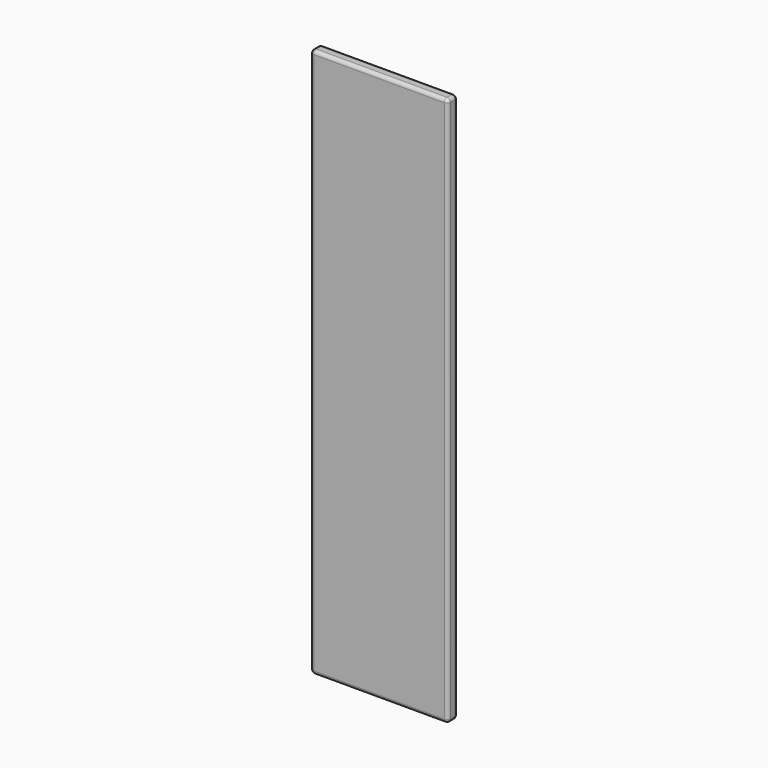
from build123d import *

# Parameters (mm, degrees)
F0_W         = 200
F0_H         = 800
F1_DEPTH     = 18
F2_R         = 5
F3_T1_DEPTH  = 8
F3_S5_W      = 5
F3_S5_H      = 5
F3_T6_DEPTH  = 5
F3_S11_W     = 5
F3_S11_H     = 5
F3_T12_DEPTH = 5


# Not quite as in the source:
# - a fillet or chamfer that OpenCascade refuses, or shapes differently, is made with other operations: its cross-section is extruded or revolved along the edge and cut away or added


with BuildPart() as f1:
    # F0 (on Front) → F1 (new body)
    with BuildSketch(Plane.XZ):
        with Locations((-100, 169.3565798058)):
            Rectangle(F0_W, F0_H)
    extrude(amount=F1_DEPTH)

    # F2
    f2_edges = [f1.edges().sort_by_distance(p)[0] for p in [
        (-200, -18, 169.35658),
        (-200, 0, 169.35658),
        (-100, -18, -230.64342),
        (-100, 0, -230.64342),
        (0, -18, 169.35658),
        (-200, -9, -230.64342),
        (0, -9, -230.64342),
        (-200, -9, 569.35658),
        (-100, -18, 569.35658),
        (-100, 0, 569.35658),
        (0, 0, 169.35658),
    ]]
    fillet(f2_edges, radius=F2_R)

    # F3: fillet of radius 5 on 1 edges, made by hand

    # F3_s2 → F3_t1 (cut)
    with BuildSketch(Plane.XZ.offset(5)):
        with BuildLine():
            ThreePointArc((0, 564.3565798058), (-1.4644660941, 567.8921137117), (-5, 569.3565798058))
            Line((-5, 569.3565798058), (0, 569.3565798058))
            Line((0, 569.3565798058), (0, 564.3565798058))
        make_face()
    extrude(amount=F3_T1_DEPTH, mode=Mode.SUBTRACT)


with BuildPart() as f3_tool4:
    # F3_s5 → F3_t6 (new body)
    with BuildSketch(Plane.YZ.offset(-5)):
        with Locations((-2.5, 566.8565798058)):
            Rectangle(F3_S5_W, F3_S5_H)
    extrude(amount=F3_T6_DEPTH)

    # F3_s7 → F3_t8 (revolve, cut)
    with BuildSketch(Plane(origin=(-5, -5, 564.3565798058), x_dir=(0, -0.7071067812, -0.7071067812), z_dir=(0, -0.7071067812, 0.7071067812))):
        with BuildLine():
            ThreePointArc((0, -5), (5, 0), (0, 5))
            Line((0, 5), (0, -5))
        make_face()
    revolve(axis=Axis((-5, -5, 564.3565798058), (1, 0, 0)), mode=Mode.SUBTRACT)


with BuildPart() as f1_1:
    add(f1.part)

    # F3_t3: cut F3_tool4
    add(f3_tool4.part, mode=Mode.SUBTRACT)


with BuildPart() as f3_tool10:
    # F3_s11 → F3_t12 (new body)
    with BuildSketch(Plane.YZ.offset(-5)):
        with Locations((-15.5, 566.8565798058)):
            Rectangle(F3_S11_W, F3_S11_H)
    extrude(amount=F3_T12_DEPTH)

    # F3_s13 → F3_t14 (revolve, cut)
    with BuildSketch(Plane(origin=(-5, -13, 564.3565798058), x_dir=(0, 0.7071067812, -0.7071067812), z_dir=(0, -0.7071067812, -0.7071067812))):
        with BuildLine():
            ThreePointArc((0, -5), (5, 0), (0, 5))
            Line((0, 5), (0, -5))
        make_face()
    revolve(axis=Axis((-5, -13, 564.3565798058), (1, 0, 0)), mode=Mode.SUBTRACT)


with BuildPart() as f1_2:
    add(f1_1.part)

    # F3_t9: cut F3_tool10
    add(f3_tool10.part, mode=Mode.SUBTRACT)


solid = f1_2.part
